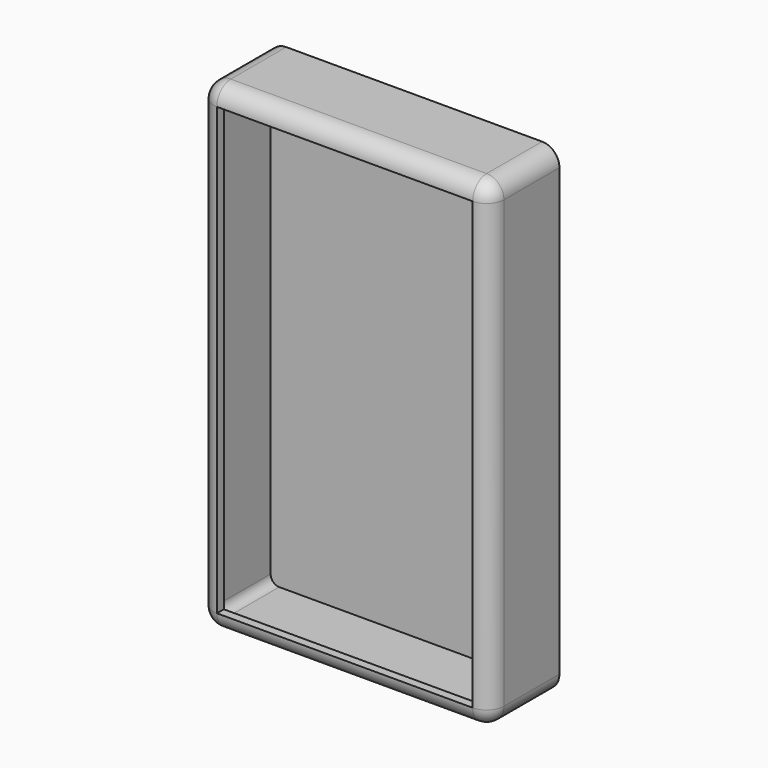
from build123d import *

# Parameters (mm, degrees)
F0_W     = 85.1108208299
F0_H     = 140.7826244831
F1_DEPTH = 25.4
F2_R     = 5.08
F3_T     = -2.54


# Not quite as in the source:
# - a shell that OpenCascade refuses in one call is made with other operations: the cavity is built on its own and cut out


with BuildPart() as f1:
    # F0 (on Front) → F1 (new body)
    with BuildSketch(Plane.XZ):
        Rectangle(F0_W, F0_H)
    extrude(amount=F1_DEPTH)

    # F2
    f2_edges = [f1.edges().sort_by_distance(p)[0] for p in [
        (0, -25.4, 70.391312),
        (-42.55541, -25.4, 0),
        (0, -25.4, -70.391312),
        (42.55541, -25.4, 0),
        (-42.55541, -12.7, 70.391312),
        (42.55541, -12.7, 70.391312),
        (-42.55541, -12.7, -70.391312),
        (42.55541, -12.7, -70.391312),
    ]]
    fillet(f2_edges, radius=F2_R)

    # F3: a shell. OpenCascade refuses it in one call, so the cavity is built on its own and cut out:
    # the body offset inwards by the wall thickness, plus a prism from it out through each open face.
    f3_core = offset(f1.part, amount=F3_T, mode=Mode.PRIVATE)
    f3_exits = [f3_core.faces().sort_by_distance(p)[0] for p in [
        (0, -22.86, 0),
    ]]
    add(f3_core, mode=Mode.SUBTRACT)
    extrude(f3_exits, amount=-F3_T, mode=Mode.SUBTRACT)


solid = f1.part
